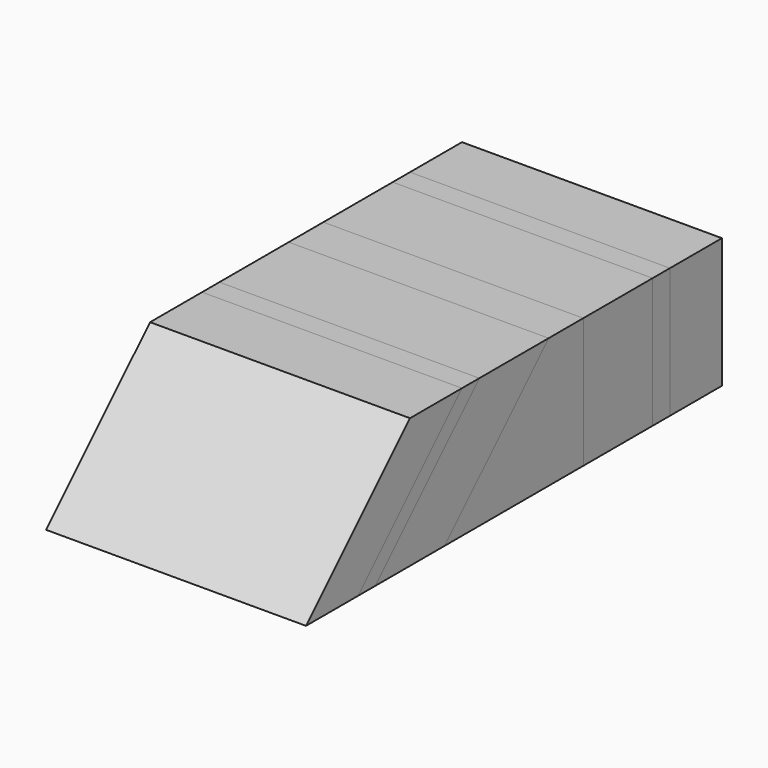
from build123d import *

# Parameters (mm, degrees)
F0_W     = 125
F0_H     = 62.5
F1_DEPTH = 125
F2_DEPTH = 62.5
F3_DEPTH = 93.75
F4_DEPTH = 31.25
F5_DEPTH = 83.3333333333
F6_DEPTH = 41.6666666667
F7_SIZE2 = 62.49999
F7_SIZE  = 62.49999
F8_SIZE  = 62.49999
F9_SIZE  = 62.49999
F10_SIZE = 62.49999
F11_SIZE = 62.49999
F12_SIZE = 62.49999


# Not quite as in the source:
# - a fillet or chamfer is up to 0.001 mm smaller than in the source, because OpenCascade refuses the exact size


with BuildPart() as f1:
    # F0 (on Front) → F1 (new body, symmetric)
    with BuildSketch(Plane.XZ):
        Rectangle(F0_W, F0_H)
    extrude(amount=F1_DEPTH, both=True)

    # F7 (size 62.5 and 62.5 in the source; OpenCascade refuses exactly that, so slightly less here)
    f7_edges = [f1.edges().sort_by_distance(p)[0] for p in [
        (0, -125, 31.25),
    ]]
    chamfer(f7_edges, length=F7_SIZE, length2=F7_SIZE2)


with BuildPart() as f2:
    # F0 (on Front) → F2 (new body, symmetric)
    with BuildSketch(Plane.XZ):
        Rectangle(F0_W, F0_H)
    extrude(amount=F2_DEPTH, both=True)

    # F8 (size 62.5 in the source; OpenCascade refuses exactly that, so slightly less here)
    f8_edges = [f2.edges().sort_by_distance(p)[0] for p in [
        (0, -62.5, 31.25),
    ]]
    chamfer(f8_edges, length=F8_SIZE)


with BuildPart() as f3:
    # F0 (on Front) → F3 (new body, symmetric)
    with BuildSketch(Plane.XZ):
        Rectangle(F0_W, F0_H)
    extrude(amount=F3_DEPTH, both=True)

    # F9 (size 62.5 in the source; OpenCascade refuses exactly that, so slightly less here)
    f9_edges = [f3.edges().sort_by_distance(p)[0] for p in [
        (0, -93.75, 31.25),
    ]]
    chamfer(f9_edges, length=F9_SIZE)


with BuildPart() as f4:
    # F0 (on Front) → F4 (new body, symmetric)
    with BuildSketch(Plane.XZ):
        Rectangle(F0_W, F0_H)
    extrude(amount=F4_DEPTH, both=True)

    # F11 (size 62.5 in the source; OpenCascade refuses exactly that, so slightly less here)
    f11_edges = [f4.edges().sort_by_distance(p)[0] for p in [
        (0, -31.25, 31.25),
    ]]
    chamfer(f11_edges, length=F11_SIZE)


with BuildPart() as f5:
    # F0 (on Front) → F5 (new body, symmetric)
    with BuildSketch(Plane.XZ):
        Rectangle(F0_W, F0_H)
    extrude(amount=F5_DEPTH, both=True)

    # F10 (size 62.5 in the source; OpenCascade refuses exactly that, so slightly less here)
    f10_edges = [f5.edges().sort_by_distance(p)[0] for p in [
        (0, -83.333333, 31.25),
    ]]
    chamfer(f10_edges, length=F10_SIZE)


with BuildPart() as f6:
    # F0 (on Front) → F6 (new body, symmetric)
    with BuildSketch(Plane.XZ):
        Rectangle(F0_W, F0_H)
    extrude(amount=F6_DEPTH, both=True)

    # F12 (size 62.5 in the source; OpenCascade refuses exactly that, so slightly less here)
    f12_edges = [f6.edges().sort_by_distance(p)[0] for p in [
        (0, -41.666667, 31.25),
    ]]
    chamfer(f12_edges, length=F12_SIZE)


solid = Compound([f1.part, f2.part, f3.part, f4.part, f5.part, f6.part])
